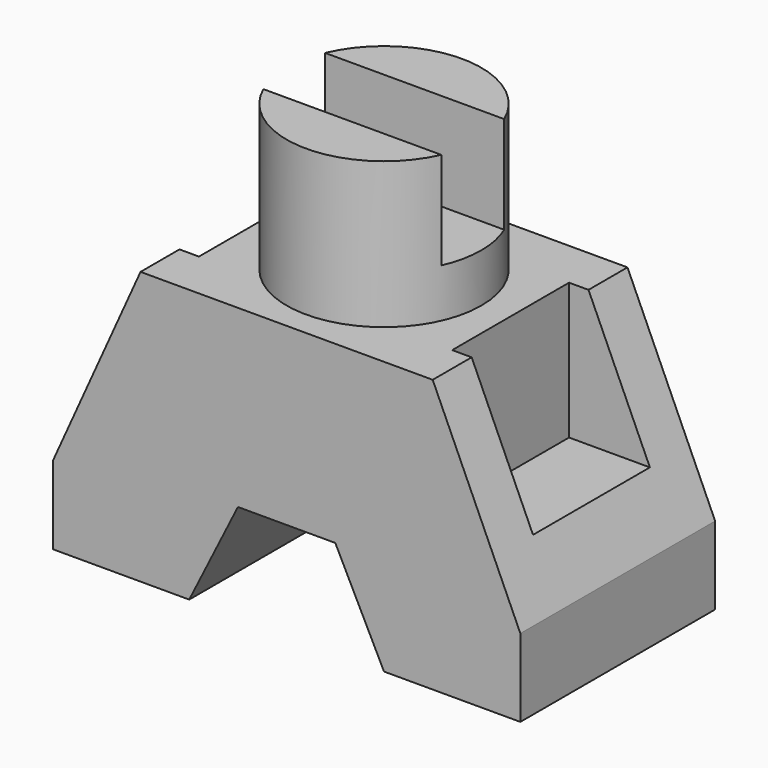
from build123d import *

# Parameters (mm, degrees)
F1_DEPTH  = 25
F3_W      = 2
F3_H      = 15
F3_W_2    = 5.2175602431
F4_DEPTH  = 14
F5_W      = 6.9340183245
F5_H      = 15
F5_W_2    = 2
F6_DEPTH  = 14
F7_R      = 10
F8_DEPTH  = 15
F10_DEPTH = 10


with BuildPart() as f1:
    # F0 (on Front) → F1 (new body)
    with BuildSketch(Plane.XZ):
        Polygon((10, -28), (24, -28), (24, -20), (15, 0), (-15, 0), (-24, -20), (-24, -28), (-10, -28), (-5, -18), (5, -18), align=None)
    extrude(amount=F1_DEPTH)

    # F3 (on face) → F4 (cut)
    with BuildSketch(Plane.XY):
        with Locations((-14, -12.5)):
            Rectangle(F3_W, F3_H)
        with Locations((-17.6087801216, -12.5)):
            Rectangle(F3_W_2, F3_H)
    extrude(amount=-F4_DEPTH, mode=Mode.SUBTRACT)

    # F5 (on face) → F6 (cut)
    with BuildSketch(Plane.XY):
        with Locations((18.4670091623, -12.5)):
            Rectangle(F5_W, F5_H)
        with Locations((14, -12.5)):
            Rectangle(F5_W_2, F5_H)
    extrude(amount=-F6_DEPTH, mode=Mode.SUBTRACT)

    # F7 (on face) → F8 (join)
    with BuildSketch(Plane.XY):
        with Locations((0, -12.5)):
            Circle(F7_R)
    extrude(amount=F8_DEPTH)

    # F9 (on face) → F10 (cut)
    with BuildSketch(Plane.XY.offset(15)):
        with BuildLine():
            Line((9.1950891808, -8.5693085904), (-9.1950891808, -8.5693085904))
            ThreePointArc((-9.1950891808, -8.5693085904), (-9.79670587, -10.4938708676), (-10, -12.5))
            ThreePointArc((-10, -12.5), (-9.7812549358, -14.5801566962), (-9.1345896238, -16.5693085904))
            Line((-9.1345896238, -16.5693085904), (9.1345896238, -16.5693085904))
            ThreePointArc((9.1345896238, -16.5693085904), (9.7812549358, -14.5801566962), (10, -12.5))
            ThreePointArc((10, -12.5), (9.79670587, -10.4938708676), (9.1950891808, -8.5693085904))
        make_face()
        with BuildLine():
            Line((10, -8.5693085904), (9.1950891808, -8.5693085904))
            ThreePointArc((9.1950891808, -8.5693085904), (9.79670587, -10.4938708676), (10, -12.5))
            Line((10, -12.5), (10, -8.5693085904))
        make_face()
    extrude(amount=-F10_DEPTH, mode=Mode.SUBTRACT)


solid = f1.part
